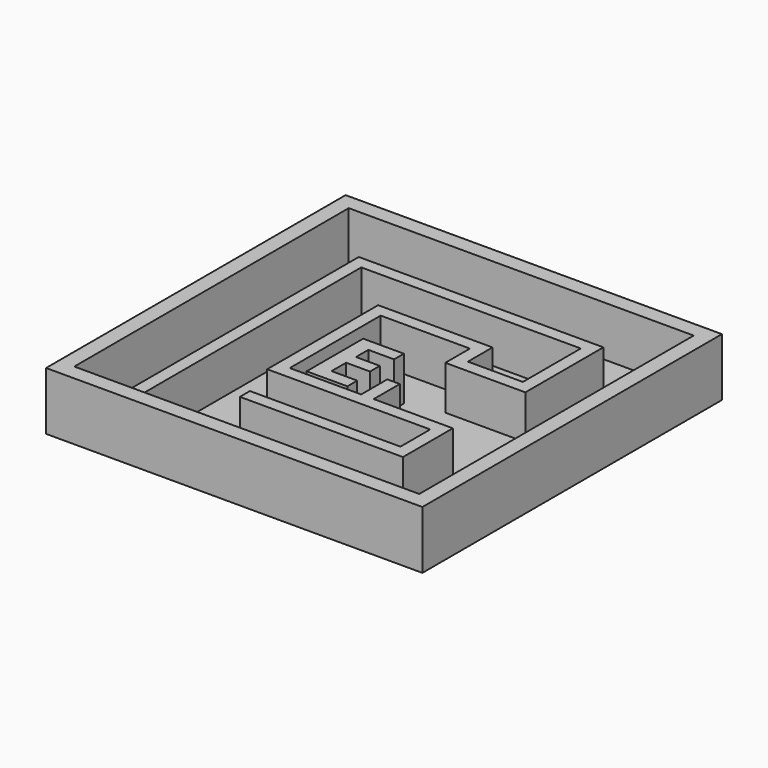
from build123d import *

# Parameters (mm, degrees)
F0_W         = 38.1
F0_H         = 37.9066020171
F1_DEPTH     = 0.79375
F2_W         = 38.1
F2_H         = 37.9066020171
F2_W_2       = 34.925
F2_H_2       = 34.7316020171
F3_DEPTH     = 5.08
F7_DEPTH     = 4.445
F8_TEXT_SIZE = 10.0214648733
F9_DEPTH     = 4.445
F5_R         = 1.27
F10_DEPTH    = 0.396875
F6_R         = 1.27
F11_DEPTH    = 0.396875


# Not quite as in the source:
# - Text() gives the source's letters only with a copy of the font that has no kerning and outlines rounded to 1/6400 em; it was checked with that copy


with BuildPart() as f1:
    # F0 (on Top) → F1 (new body)
    with BuildSketch(Plane.XY):
        with Locations((-49.0613915026, -5.5621918291)):
            Rectangle(F0_W, F0_H)
    extrude(amount=F1_DEPTH)

    # F2 (on face) → F3 (join)
    with BuildSketch(Plane.XY.offset(0.79375)):
        with Locations((-49.0613915026, -5.5621918291)):
            Rectangle(F2_W, F2_H)
        with Locations((-49.0613915026, -5.5621918291)):
            Rectangle(F2_W_2, F2_H_2, mode=Mode.SUBTRACT)
    extrude(amount=F3_DEPTH)

    # F4 (on face) → F7 (join)
    with BuildSketch(Plane.XY.offset(0.79375)):
        Polygon((-61.4438915026, 6.7236091795), (-61.4438915026, -22.9279928376), (-60.1738915026, -22.9279928376), (-60.1738915026, 5.4536091795), (-37.9488915026, 5.4536091795), (-37.9488915026, -1.8816381059), (-43.5132453561, -1.8816381059), (-43.5132453561, 1.2361826077), (-44.7832453561, 1.2361826077), (-55.0938915026, 1.2361826077), (-55.0938915026, -0.0338173923), (-55.0938915026, -11.5367079931), (-55.0938915026, -12.8067079931), (-48.5916206956, -12.8067079931), (-38.5838915026, -12.8067079931), (-38.5838915026, -16.5779928376), (-53.8238915026, -16.5779928376), (-53.8238915026, -17.8479928376), (-38.5838915026, -17.8479928376), (-37.3138915026, -17.8479928376), (-37.3138915026, -12.8067079931), (-37.3138915026, -11.5367079931), (-45.3236725688, -11.5367079931), (-45.3236725688, -8.2316381059), (-46.5936725688, -8.2316381059), (-46.5936725688, -11.5367079931), (-53.8238915026, -11.5367079931), (-53.8238915026, -0.0338173923), (-44.7832453561, -0.0338173923), (-44.7832453561, -3.1516381059), (-43.5132453561, -3.1516381059), (-37.9488915026, -3.1516381059), (-36.6788915026, -3.1516381059), (-36.6788915026, 6.7236091795), (-37.9488915026, 6.7236091795), (-60.1738915026, 6.7236091795), align=None)
    extrude(amount=F7_DEPTH)

    # F8 (on face) → F9 (join)
    with BuildSketch(Plane.XY.offset(0.79375)):
        with Locations((-53.3358119428, -11.134814471)):
            Text('E', F8_TEXT_SIZE, font='Open Sans', font_style=FontStyle.BOLD, text_align=(TextAlign.LEFT, TextAlign.BOTTOM))
    extrude(amount=F9_DEPTH)

    # F5 (on face) → F10 (cut)
    with BuildSketch(Plane.XY.offset(0.79375)):
        with Locations((-63.9573261142, -18.397340551)):
            Circle(F5_R)
    extrude(amount=-F10_DEPTH, mode=Mode.SUBTRACT)

    # F6 (on face) → F11 (cut)
    with BuildSketch(Plane.XY.offset(0.79375)):
        with Locations((-40.5282483102, 1.0310473011)):
            Circle(F6_R)
    extrude(amount=-F11_DEPTH, mode=Mode.SUBTRACT)


solid = f1.part
